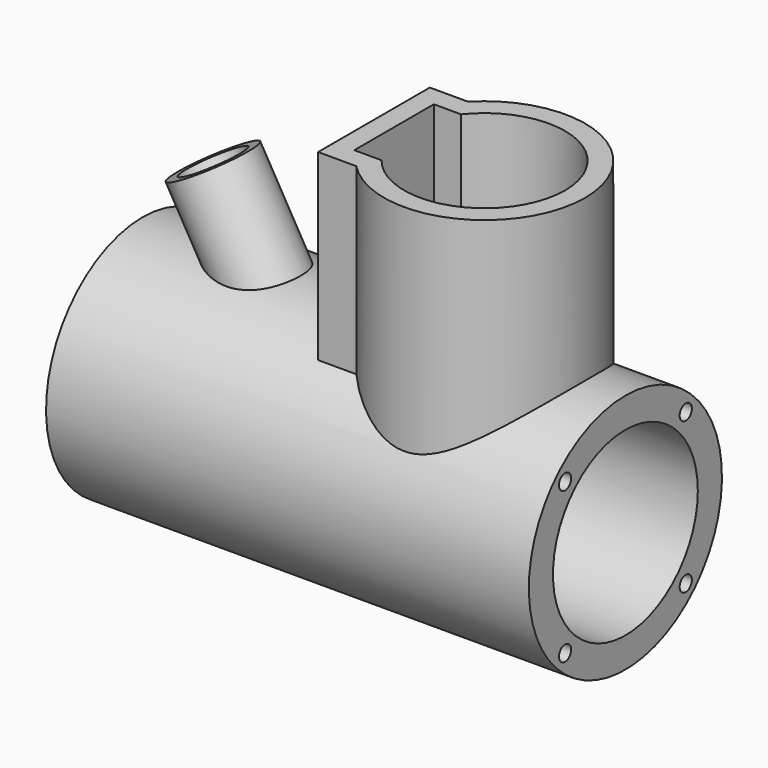
from build123d import *

# Parameters (mm, degrees)
F0_W      = 152.4
F0_H      = 38.1
F3_R      = 31.75
F4_DEPTH  = 25.4
F5_DEPTH  = 50.8
F7_DEPTH  = 76.2
F11_DEPTH = 76.2
F12_R     = 28.575
F13_DEPTH = 146.05
F14_R     = 9.525
F15_DEPTH = 50.8
F17_D     = 4.826
F17_DEPTH = 12.7
F17_TIP   = 1.4498766737
F19_D     = 12.7
F19_DEPTH = 12.7
F19_TIP   = 3.8154649308


# Not quite as in the source:
# - a feature names something its author has since deleted; it is built from what else it names


with BuildPart() as f1:
    # F0 (on Front) → F1 (revolve)
    with BuildSketch(Plane.XZ):
        with Locations((76.2, 19.05)):
            Rectangle(F0_W, F0_H)
    revolve(axis=Axis((76.2, 0, 0), (1, 0, 0)))

    # F3 (on offset) → F4 (join)
    with BuildSketch(Plane.XY.offset(38.1)):
        with Locations((107.95, 0)):
            Circle(F3_R)
    extrude(amount=-F4_DEPTH)

    # F5 (add): a face of the model
    f5_faces = [f1.faces().sort_by_distance(p)[0] for p in [
        (107.95, 0, 38.1),
    ]]
    extrude(f5_faces, amount=F5_DEPTH)

    # F6 (on face) → F7 (join)
    with BuildSketch(Plane.XY.offset(88.9)):
        with BuildLine():
            Line((73.025, -22.0412760045), (85.097327244, -22.0412760045))
            ThreePointArc((85.097327244, -22.0412760045), (76.2, 0), (85.097327244, 22.0412760045))
            Line((85.097327244, 22.0412760045), (73.025, 22.0412760045))
            Line((73.025, 22.0412760045), (73.025, -22.0412760045))
        make_face()
    extrude(amount=-F7_DEPTH)

    # F8 (on Front) → F9 (revolve)
    with BuildSketch(Plane.XZ):
        Polygon((33.2235226281, 67.1248349075), (22.225, 60.7748349075), (38.982496247, 31.75), (49.9810188751, 38.1), align=None)
    revolve(axis=Axis((30.6037481235, 0, 46.2624174538), (0.5, 0, -0.8660254038)))

    # F10 (on face) → F11 (cut)
    with BuildSketch(Plane.XY.offset(88.9)):
        with BuildLine():
            Line((79.3750002146, -15.69127579), (87.9764211223, -15.69127579))
            ThreePointArc((87.9764211223, -15.69127579), (133.3499997854, 0), (87.9764211223, 15.69127579))
            Line((87.9764211223, 15.69127579), (79.3750002146, 15.69127579))
            Line((79.3750002146, 15.69127579), (79.3750002146, -15.69127579))
        make_face()
    extrude(amount=-F11_DEPTH, mode=Mode.SUBTRACT)

    # F12 (on face) → F13 (cut)
    with BuildSketch(Plane.YZ.offset(152.4)):
        Circle(F12_R)
    extrude(amount=-F13_DEPTH, mode=Mode.SUBTRACT)

    # F14 (on face) → F15 (cut)
    with BuildSketch(Plane(origin=(-20.7600254704, 0, 35.9574188811), x_dir=(0.8660254038, 0, 0.5), z_dir=(-0.5, 0, 0.8660254038))):
        with Locations((49.6348320529, 0)):
            Circle(F14_R)
    extrude(amount=-F15_DEPTH, mode=Mode.SUBTRACT)

    # F17
    with Locations(Plane.YZ.offset(152.4)):
        with Locations((-23.8125, 23.8125), (23.8125, 23.8125), (23.8125, -23.8125), (-23.8125, -23.8125)):
            Hole(F17_D / 2, depth=F17_DEPTH)
            with Locations((0, 0, -(F17_DEPTH + F17_TIP / 2))):  # 118° drill point
                Cone(0, F17_D / 2, F17_TIP, mode=Mode.SUBTRACT)

    # F19
    with Locations(Plane(origin=(0, 0, 0), x_dir=(0, -1, 0), z_dir=(-1, 0, 0))):
        with Locations((0, 0)):
            Hole(F19_D / 2, depth=F19_DEPTH)
            with Locations((0, 0, -(F19_DEPTH + F19_TIP / 2))):  # 118° drill point
                Cone(0, F19_D / 2, F19_TIP, mode=Mode.SUBTRACT)


solid = f1.part
